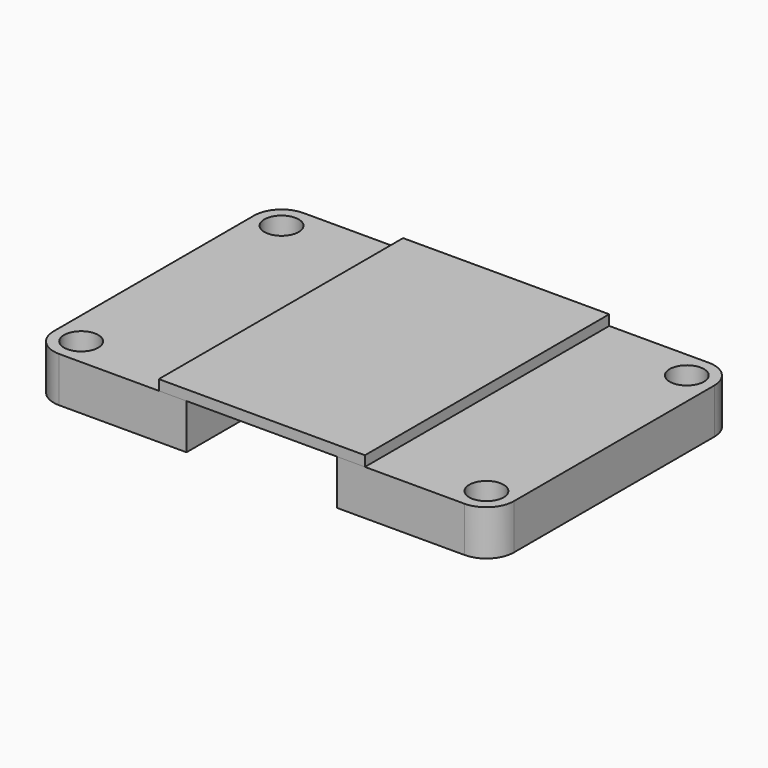
from build123d import *

# Parameters (mm, degrees)
F0_R     = 5
F1_DEPTH = 13.16
F2_W     = 8.08
F2_H     = 89
F3_DEPTH = 3
F4_DEPTH = 170


# Not quite as in the source:
# - an extrude ends at something that could not be found from the text; its depth is read off the source's solid


with BuildPart() as f1:
    # F0 (on Top) → F1 (new body)
    with BuildSketch(Plane.XY):
        with BuildLine():
            Line((-59.06, -44.5), (-21.96, -44.5))
            Line((-21.96, -44.5), (-21.96, 44.5))
            Line((-21.96, 44.5), (-59.06, 44.5))
            ThreePointArc((-59.06, 44.5), (-64.7168542495, 42.1568542495), (-67.06, 36.5))
            Line((-67.06, 36.5), (-67.06, -36.5))
            ThreePointArc((-67.06, -36.5), (-64.7168542495, -42.1568542495), (-59.06, -44.5))
        make_face()
        with Locations((-59.06, -36.5)):
            Circle(F0_R, mode=Mode.SUBTRACT)
        with Locations((-59.06, 36.5)):
            Circle(F0_R, mode=Mode.SUBTRACT)
    extrude(amount=F1_DEPTH)

    # F0 (on Top) → F4 (cut, through all)
    with BuildSketch(Plane.XY):
        with Locations((59.06, -36.5)):
            Circle(F0_R)
        with Locations((-59.06, -36.5)):
            Circle(F0_R)
        with Locations((-59.06, 36.5)):
            Circle(F0_R)
        with Locations((59.06, 36.5)):
            Circle(F0_R)
    extrude(amount=-F4_DEPTH, mode=Mode.SUBTRACT)


with BuildPart() as f1b:
    # F0 (on Top) → F1, piece 2 (new body)
    with BuildSketch(Plane.XY):
        with BuildLine():
            Line((21.94, -44.5), (59.06, -44.5))
            ThreePointArc((59.06, -44.5), (64.7168542495, -42.1568542495), (67.06, -36.5))
            Line((67.06, -36.5), (67.06, 36.5))
            ThreePointArc((67.06, 36.5), (64.7168542495, 42.1568542495), (59.06, 44.5))
            Line((59.06, 44.5), (21.94, 44.5))
            Line((21.94, 44.5), (21.94, -44.5))
        make_face()
        with Locations((59.06, -36.5)):
            Circle(F0_R, mode=Mode.SUBTRACT)
        with Locations((59.06, 36.5)):
            Circle(F0_R, mode=Mode.SUBTRACT)
    extrude(amount=F1_DEPTH)


with BuildPart() as f3:
    # F2 (on face) → F3 (new body)
    with BuildSketch(Plane.XY.offset(13.16)):
        Polygon((30.04, 44.5), (0, 44.5), (-21.96, 44.5), (-21.96, -44.5), (30.04, -44.5), align=None)
        with Locations((-26, 0)):
            Rectangle(F2_W, F2_H)
    extrude(amount=F3_DEPTH)


solid = Compound([f1.part, f1b.part, f3.part])
